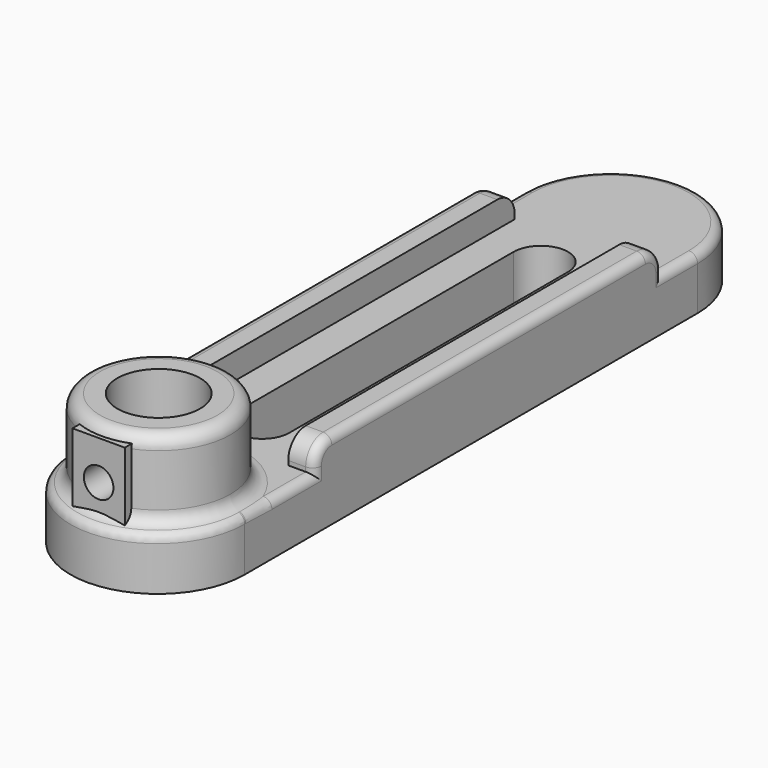
from build123d import *

# Parameters (mm, degrees)
F0_R          = 12.5
F1_DEPTH      = 12
F3_START      = 12
F2_R          = 16.5
F2_R_2        = 12.5
F2_R_3        = 9.5
F3_DEPTH      = 18
F4_DEPTH      = 30
F5_R          = 9.5
F6_DEPTH      = 25
F6_DEPTH_BACK = 100
F7_R          = 3
F9_DEPTH      = 50
F9_DEPTH_BACK = 50
F10_R         = 5
F11_R         = 19.99999
F12_W         = 12
F12_H         = 6
F13_DEPTH     = 28
F15_START     = 70
F14_R         = 3.4
F15_DEPTH     = 30
F16_R         = 2


# Not quite as in the source:
# - a fillet or chamfer is up to 0.001 mm smaller than in the source, because OpenCascade refuses the exact size


with BuildPart() as f1:
    # F0 (on Top) → F1 (new body)
    with BuildSketch(Plane.XY):
        with BuildLine():
            Line((20, -70), (20, 80))
            Line((20, 80), (-20, 80))
            Line((-20, 80), (-20, -70))
            ThreePointArc((-20, -70), (0, -90), (20, -70))
        make_face()
        with Locations((0, -70)):
            Circle(F0_R, mode=Mode.SUBTRACT)
        with BuildLine():
            ThreePointArc((6.2482987692, -40.1458166336), (-0.0729132787, -46.2495746778), (-6.25, -40))
            Line((-6.25, -40), (-6.25, 40))
            ThreePointArc((-6.25, 40), (-0.0729132787, 46.2495746778), (6.2482987692, 40.1458166336))
            ThreePointArc((6.2482987692, 40.1458166336), (6.25, 40), (6.2482987692, 39.8541833664))
            Line((6.2482987692, 39.8541833664), (6.2482987692, -39.8541833664))
            ThreePointArc((6.2482987692, -39.8541833664), (6.25, -40), (6.2482987692, -40.1458166336))
        make_face(mode=Mode.SUBTRACT)
    extrude(amount=F1_DEPTH)

    # F2 (on Top) → F3 (join)
    with BuildSketch(Plane.XY.offset(F3_START)):
        with Locations((0, -69.6852505207)):
            Circle(F2_R)
        with Locations((0, -69.6852505207)):
            Circle(F2_R_2, mode=Mode.SUBTRACT)
        with Locations((0, -69.6852505207)):
            Circle(F2_R_2)
        with Locations((0, -69.6852505207)):
            Circle(F2_R_3, mode=Mode.SUBTRACT)
    extrude(amount=F3_DEPTH)

    # F2 (on Top) → F4 (join)
    with BuildSketch(Plane.XY):
        with Locations((0, -69.6852505207)):
            Circle(F2_R_2)
        with Locations((0, -69.6852505207)):
            Circle(F2_R_3, mode=Mode.SUBTRACT)
        with Locations((0, -69.6852505207)):
            Circle(F2_R_3)
    extrude(amount=F4_DEPTH)

    # F5 (on Top) → F6 (cut, two sides)
    with BuildSketch(Plane.XY) as f6_sk:
        with Locations((0, -69.6852505207)):
            Circle(F5_R)
    extrude(amount=-F6_DEPTH, mode=Mode.SUBTRACT)
    extrude(f6_sk.sketch, amount=F6_DEPTH_BACK, mode=Mode.SUBTRACT)

    # F7
    f7_edges = [f1.edges().sort_by_distance(p)[0] for p in [
        (-16.5, -69.685251, 30),
        (-16.5, -69.685251, 12),
    ]]
    fillet(f7_edges, radius=F7_R)

    # F8 (on Front) → F9 (join, two sides)
    with BuildSketch(Plane.XZ) as f9_sk:
        Polygon((14, 0), (20, 0), (20, 18), (14, 18), (14, 12), align=None)
        Polygon((-14, 0), (-14, 12), (-14, 18), (-20, 18), (-20, 0), align=None)
    extrude(amount=F9_DEPTH)
    extrude(f9_sk.sketch, amount=-F9_DEPTH_BACK)

    # F10
    f10_edges = [f1.edges().sort_by_distance(p)[0] for p in [
        (17, 50, 18),
        (-17, 50, 18),
        (-17, -50, 18),
        (17, -50, 18),
    ]]
    fillet(f10_edges, radius=F10_R)

    # F11 (radius 20 in the source; OpenCascade refuses exactly that, so slightly less here)
    f11_edges = [f1.edges().sort_by_distance(p)[0] for p in [
        (-20, 80, 6),
        (20, 80, 6),
    ]]
    fillet(f11_edges, radius=F11_R)

    # F12 (on Top) → F13 (join)
    with BuildSketch(Plane.XY):
        with Locations((0, -83.9288532734)):
            Rectangle(F12_W, F12_H)
    extrude(amount=F13_DEPTH)

    # F14 (on Front) → F15 (cut)
    with BuildSketch(Plane.XZ.offset(F15_START)):
        with Locations((0, 19)):
            Circle(F14_R)
    extrude(amount=F15_DEPTH, mode=Mode.SUBTRACT)

    # F16
    f16_edges = [f1.edges().sort_by_distance(p)[0] for p in [
        (20, 55.000005, 12),
        (-14.142139, 74.142139, 12),
        (-20, 55.000005, 12),
        (20, -60, 12),
        (-20, -48.535534, 16.535534),
        (-20, 0, 18),
        (20, 0, 18),
        (20, -48.535534, 16.535534),
    ]]
    fillet(f16_edges, radius=F16_R)


solid = f1.part
